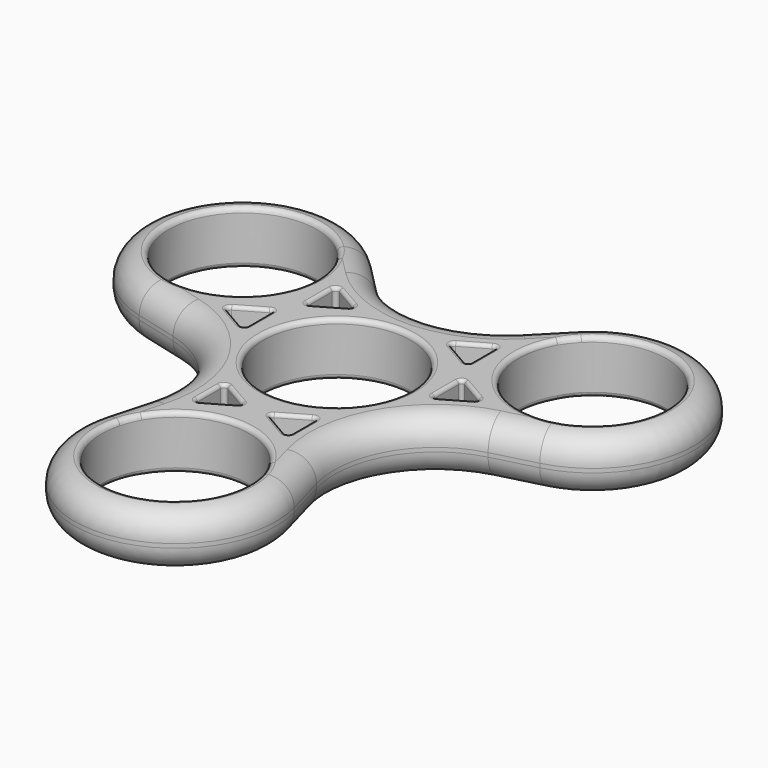
from build123d import *

# Parameters (mm, degrees)
F0_R     = 5.5
F1_DEPTH = 4
F2_R     = 1.85
F3_R     = 0.35
F5_DEPTH = 4
F6_R     = 0.25


# Not quite as in the source:
# - a feature names something its author has since deleted; it is built from what else it names


with BuildPart() as f1:
    # F0 (on Top) → F1 (new body)
    with BuildSketch(Plane.XY):
        with BuildLine():
            Line((-5.3430418424, 10.42403323), (-7.6473392144, 12.7632598141))
            ThreePointArc((-7.6473392144, 12.7632598141), (-19.4855715851, 11.25), (-14.8769768413, 0.241160124))
            Line((-14.8769768413, 0.241160124), (-11.6989985083, -0.584806646))
            ThreePointArc((-11.6989985083, -0.584806646), (-7.0904037644, -4.093646522), (-6.3559566659, -9.839226584))
            Line((-6.3559566659, -9.839226584), (-7.2296376269, -13.004419938))
            ThreePointArc((-7.2296376269, -13.004419938), (0, -22.5), (7.2296376269, -13.004419938))
            Line((7.2296376269, -13.004419938), (6.3559566659, -9.839226584))
            ThreePointArc((6.3559566659, -9.839226584), (7.0904037644, -4.093646522), (11.6989985083, -0.584806646))
            Line((11.6989985083, -0.584806646), (14.8769768413, 0.241160124))
            ThreePointArc((14.8769768413, 0.241160124), (19.4855715851, 11.25), (7.6473392144, 12.7632598141))
            Line((7.6473392144, 12.7632598141), (5.3430418424, 10.42403323))
            ThreePointArc((5.3430418424, 10.42403323), (0, 8.1872930441), (-5.3430418424, 10.42403323))
        make_face()
        with Locations((0, -15)):
            Circle(F0_R, mode=Mode.SUBTRACT)
        with Locations((-12.9903810568, 7.5)):
            Circle(F0_R, mode=Mode.SUBTRACT)
        Circle(F0_R, mode=Mode.SUBTRACT)
        with Locations((12.9903810568, 7.5)):
            Circle(F0_R, mode=Mode.SUBTRACT)
    extrude(amount=F1_DEPTH)

    # F2
    f2_edges = [f1.edges().sort_by_distance(p)[0] for p in [
        (6.355957, -9.839227, 2),
        (11.698999, -0.584807, 2),
        (7.090404, -4.093647, 0),
        (7.090404, -4.093647, 4),
        (-7.229638, -13.00442, 2),
        (7.229638, -13.00442, 2),
        (0, -22.5, 0),
        (0, -22.5, 4),
        (6.792797, -11.421823, 0),
        (6.792797, -11.421823, 4),
        (14.876977, 0.24116, 2),
        (7.647339, 12.76326, 2),
        (19.485572, 11.25, 0),
        (19.485572, 11.25, 4),
        (13.287988, -0.171823, 0),
        (13.287988, -0.171823, 4),
        (-11.698999, -0.584807, 2),
        (-6.355957, -9.839227, 2),
        (-7.090404, -4.093647, 0),
        (-7.090404, -4.093647, 4),
        (-6.792797, -11.421823, 0),
        (-6.792797, -11.421823, 4),
        (-7.647339, 12.76326, 2),
        (-14.876977, 0.24116, 2),
        (-19.485572, 11.25, 0),
        (-19.485572, 11.25, 4),
        (-13.287988, -0.171823, 0),
        (-13.287988, -0.171823, 4),
        (-5.343042, 10.424033, 2),
        (-6.495191, 11.593647, 0),
        (-6.495191, 11.593647, 4),
        (5.343042, 10.424033, 2),
        (0, 8.187293, 0),
        (0, 8.187293, 4),
        (6.495191, 11.593647, 0),
        (6.495191, 11.593647, 4),
    ]]
    fillet(f2_edges, radius=F2_R)

    # F3
    f3_edges = [f1.edges().sort_by_distance(p)[0] for p in [
        (5.5, 0, 2),
        (-5.5, 0, 0),
        (-5.5, 0, 4),
        (5.5, -15, 2),
        (-5.5, -15, 0),
        (-5.5, -15, 4),
        (18.490381, 7.5, 2),
        (7.490381, 7.5, 0),
        (7.490381, 7.5, 4),
        (-7.490381, 7.5, 2),
        (-18.490381, 7.5, 0),
        (-18.490381, 7.5, 4),
    ]]
    fillet(f3_edges, radius=F3_R)

    # F4 (on face) → F5 (cut, through all)
    with BuildSketch(Plane(origin=(0, 0, 0), x_dir=(1, 0, 0), z_dir=(0, 0, -1))):
        with BuildLine():
            ThreePointArc((-3.125, 8.7834936491), (-3.375, 8.7834936491), (-3.5, 8.5669872981))
            Line((-3.5, 8.5669872981), (-3.5, 6.4330127019))
            ThreePointArc((-3.5, 6.4330127019), (-3.375, 6.2165063509), (-3.125, 6.2165063509))
            Line((-3.125, 6.2165063509), (-1.2019237886, 7.3267949192))
            ThreePointArc((-1.2019237886, 7.3267949192), (-1.1019237886, 7.5), (-1.2019237886, 7.6732050808))
            Line((-1.2019237886, 7.6732050808), (-3.125, 8.7834936491))
        make_face()
        with BuildLine():
            ThreePointArc((1.2019237886, 7.6732050808), (1.1019237886, 7.5), (1.2019237886, 7.3267949192))
            Line((1.2019237886, 7.3267949192), (3.125, 6.2165063509))
            ThreePointArc((3.125, 6.2165063509), (3.375, 6.2165063509), (3.5, 6.4330127019))
            Line((3.5, 6.4330127019), (3.5, 8.5669872981))
            ThreePointArc((3.5, 8.5669872981), (3.375, 8.7834936491), (3.125, 8.7834936491))
            Line((3.125, 8.7834936491), (1.2019237886, 7.6732050808))
        make_face()
        with BuildLine():
            ThreePointArc((7.3211524227, -0.1854174377), (7.0711524227, -0.1854174377), (6.9461524227, -0.4019237886))
            Line((6.9461524227, -0.4019237886), (6.9461524227, -2.6225009252))
            ThreePointArc((6.9461524227, -2.6225009252), (7.0461524227, -2.795706006), (7.2461524227, -2.795706006))
            Line((7.2461524227, -2.795706006), (9.1692286341, -1.6854174377))
            ThreePointArc((9.1692286341, -1.6854174377), (9.2942286341, -1.4689110868), (9.1692286341, -1.2524047358))
            Line((9.1692286341, -1.2524047358), (7.3211524227, -0.1854174377))
        make_face()
        with BuildLine():
            ThreePointArc((3.8211524227, -5.8145825623), (3.6961524227, -6.0310889132), (3.8211524227, -6.2475952642))
            Line((3.8211524227, -6.2475952642), (5.6692286341, -7.3145825623))
            ThreePointArc((5.6692286341, -7.3145825623), (5.9192286341, -7.3145825623), (6.0442286341, -7.0980762114))
            Line((6.0442286341, -7.0980762114), (6.0442286341, -4.8774990748))
            ThreePointArc((6.0442286341, -4.8774990748), (5.9442286341, -4.704293994), (5.7442286341, -4.704293994))
            Line((5.7442286341, -4.704293994), (3.8211524227, -5.8145825623))
        make_face()
        with BuildLine():
            ThreePointArc((-3.8211524227, -6.2475952642), (-3.6961524227, -6.0310889132), (-3.8211524227, -5.8145825623))
            Line((-3.8211524227, -5.8145825623), (-5.7442286341, -4.704293994))
            ThreePointArc((-5.7442286341, -4.704293994), (-5.9442286341, -4.704293994), (-6.0442286341, -4.8774990748))
            Line((-6.0442286341, -4.8774990748), (-6.0442286341, -7.0980762114))
            ThreePointArc((-6.0442286341, -7.0980762114), (-5.9192286341, -7.3145825623), (-5.6692286341, -7.3145825623))
            Line((-5.6692286341, -7.3145825623), (-3.8211524227, -6.2475952642))
        make_face()
        with BuildLine():
            ThreePointArc((-6.9461524227, -0.4019237886), (-7.0711524227, -0.1854174377), (-7.3211524227, -0.1854174377))
            Line((-7.3211524227, -0.1854174377), (-9.1692286341, -1.2524047358))
            ThreePointArc((-9.1692286341, -1.2524047358), (-9.2942286341, -1.4689110868), (-9.1692286341, -1.6854174377))
            Line((-9.1692286341, -1.6854174377), (-7.2461524227, -2.795706006))
            ThreePointArc((-7.2461524227, -2.795706006), (-7.0461524227, -2.795706006), (-6.9461524227, -2.6225009252))
            Line((-6.9461524227, -2.6225009252), (-6.9461524227, -0.4019237886))
        make_face()
    extrude(amount=-F5_DEPTH, mode=Mode.SUBTRACT)

    # F6
    f6_edges = [f1.edges().sort_by_distance(p)[0] for p in [
        (1.201924, -7.326795, 2),
        (3.125, -6.216506, 2),
        (2.163462, -6.771651, 0),
        (2.163462, -6.771651, 4),
        (-3.125, -6.216506, 2),
        (-1.201924, -7.326795, 2),
        (-2.163462, -6.771651, 0),
        (-2.163462, -6.771651, 4),
        (-3.5, -6.433013, 2),
        (-3.375, -6.216506, 0),
        (-3.375, -6.216506, 4),
        (-3.5, -8.566987, 2),
        (-3.5, -7.5, 0),
        (-3.5, -7.5, 4),
        (-3.125, -8.783494, 2),
        (-3.375, -8.783494, 0),
        (-3.375, -8.783494, 4),
        (-1.201924, -7.673205, 2),
        (-2.163462, -8.228349, 0),
        (-2.163462, -8.228349, 4),
        (3.125, -8.783494, 2),
        (1.201924, -7.673205, 2),
        (2.163462, -8.228349, 0),
        (2.163462, -8.228349, 4),
        (3.5, -6.433013, 2),
        (3.5, -8.566987, 2),
        (3.5, -7.5, 0),
        (3.5, -7.5, 4),
        (3.375, -8.783494, 0),
        (3.375, -8.783494, 4),
        (3.375, -6.216506, 0),
        (3.375, -6.216506, 4),
        (9.169229, 1.252405, 2),
        (7.321152, 0.185417, 2),
        (8.245191, 0.718911, 0),
        (8.245191, 0.718911, 4),
        (5.744229, 4.704294, 2),
        (3.821152, 5.814583, 2),
        (4.782691, 5.259438, 0),
        (4.782691, 5.259438, 4),
        (-3.821152, 5.814583, 2),
        (-5.744229, 4.704294, 2),
        (-4.782691, 5.259438, 0),
        (-4.782691, 5.259438, 4),
        (-6.946152, 2.622501, 2),
        (-6.946152, 0.401924, 2),
        (-6.946152, 1.512212, 0),
        (-6.946152, 1.512212, 4),
    ]]
    fillet(f6_edges, radius=F6_R)


solid = f1.part
